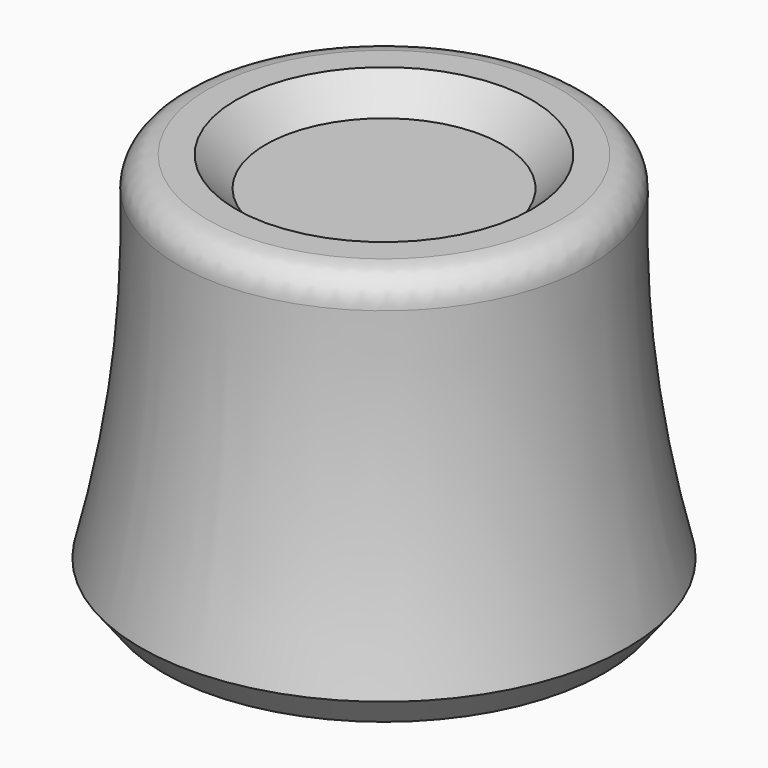
from build123d import *

# Parameters (mm, degrees)
F4_R = 1


# Not quite as in the source:
# - a fillet or chamfer that OpenCascade refuses, or shapes differently, is made with other operations: its cross-section is extruded or revolved along the edge and cut away or added


with BuildPart() as f1:
    # F0 (on Front) → F1 (revolve)
    with BuildSketch(Plane.XZ):
        with BuildLine():
            Line((0, 12), (0, 10))
            Line((0, 10), (3.1, 10))
            Line((3.1, 10), (3.1, 0))
            Line((3.1, 0), (8.5, 0))
            ThreePointArc((8.5, 0), (7.2147663015, 6.4382422656), (7, 13))
            Line((7, 13), (5, 13))
            Line((5, 13), (4, 12))
            Line((4, 12), (0, 12))
        make_face()
    revolve(axis=Axis((0, 0, 11), (0, 0, -1)))

    # F3: chamfer of 0.8 on 2 edges, made by hand

    # F3_s1 → F3_t2 (revolve, cut)
    with BuildSketch(Plane.XZ):
        Polygon((3.1, 0.8), (3.9, 0), (3.1, 0), align=None)
    revolve(axis=Axis((0, 0, 0), (0, 0, -1)), mode=Mode.SUBTRACT)

    # F3_s3 → F3_t4 (revolve, cut)
    with BuildSketch(Plane.XZ):
        with BuildLine():
            Line((7.4526927913, 0), (8.2271718294, 1.0004550311))
            ThreePointArc((8.2271718294, 1.0004550311), (8.3578103434, 0.5086375801), (8.5, 0))
            Line((8.5, 0), (7.4526927913, 0))
        make_face()
    revolve(axis=Axis((0, 0, 0), (0, 0, -1)), mode=Mode.SUBTRACT)

    # F4
    f4_edges = [f1.edges().sort_by_distance(p)[0] for p in [
        (-7, 0, 13),
    ]]
    fillet(f4_edges, radius=F4_R)


solid = f1.part
